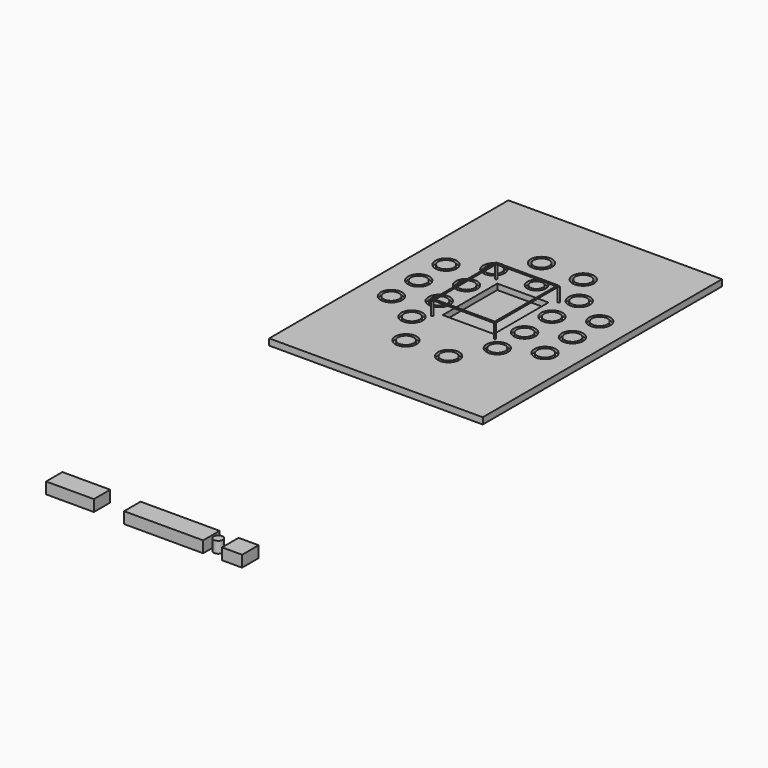
from build123d import *

# Parameters (mm, degrees)
F0_W      = 22860
F0_H      = 32004
F1_DEPTH  = 25.4
F2_W      = 5486.4
F2_H      = 7315.2
F3_DEPTH  = 76.2
F2_R      = 838.2
F4_DEPTH  = 685.8
F2_R_2    = 685.8
F2_R_3    = 844.55
F2_W_2    = 22872.7
F2_H_2    = 32016.7
F2_R_4    = 1143
F2_R_5    = 101.6
F2_R_6    = 1149.35
F2_R_7    = 990.6
F5_DEPTH  = 355.6
F6_DEPTH  = 2133.6
F8_W      = 6705.6
F8_H      = 8534.4
F8_W_2    = 6502.4
F8_H_2    = 8331.2
F9_DEPTH  = 101.6
F10_W     = 5118.2244420052
F10_H     = 2182.9090118408
F11_DEPTH = 1219.2
F10_W_2   = 8467.0696258545
F10_H_2   = 2208.8012695312
F10_W_3   = 2147.4456787109
F10_R     = 490.8447265625


# Not quite as in the source:
# - a feature names something its author has since deleted; it is built from what else it names


with BuildPart() as f1:
    # F0 (on Top) → F1 (new body)
    with BuildSketch(Plane.XY):
        with Locations((11430, 16002)):
            Rectangle(F0_W, F0_H)
    extrude(amount=F1_DEPTH)

    # F2 (on Top) → F6 (join)
    with BuildSketch(Plane.XY):
        with Locations((8077.2, 20269.2)):
            Circle(F2_R_5)
        with Locations((14782.8, 20269.2)):
            Circle(F2_R_5)
        with Locations((8077.2, 11734.8)):
            Circle(F2_R_5)
        with Locations((14782.8, 11734.8)):
            Circle(F2_R_5)
    extrude(amount=F6_DEPTH)

    # F8 (on offset) → F9 (join)
    with BuildSketch(Plane.XY.offset(2133.6)):
        with Locations((11430, 16002)):
            Rectangle(F8_W, F8_H)
        with Locations((11430, 16002)):
            Rectangle(F8_W_2, F8_H_2, mode=Mode.SUBTRACT)
    extrude(amount=F9_DEPTH)


with BuildPart() as f3:
    # F2 (on Top) → F3 (new body)
    with BuildSketch(Plane.XY):
        with Locations((11430, 16002)):
            Rectangle(F2_W, F2_H)
    extrude(amount=F3_DEPTH)


with BuildPart() as f4:
    # F2 (on Top) → F4 (new body)
    with BuildSketch(Plane.XY):
        with Locations((3200.4, 12344.4)):
            Circle(F2_R)
    extrude(amount=F4_DEPTH)


with BuildPart() as f4b:
    # F2 (on Top) → F4, piece 2 (new body)
    with BuildSketch(Plane.XY):
        with Locations((3200.4, 16002)):
            Circle(F2_R)
    extrude(amount=F4_DEPTH)


with BuildPart() as f4c:
    # F2 (on Top) → F4, piece 3 (new body)
    with BuildSketch(Plane.XY):
        with Locations((3200.4, 19659.6)):
            Circle(F2_R)
    extrude(amount=F4_DEPTH)


with BuildPart() as f4d:
    # F2 (on Top) → F4, piece 4 (new body)
    with BuildSketch(Plane.XY):
        with Locations((6858, 21488.4)):
            Circle(F2_R)
    extrude(amount=F4_DEPTH)


with BuildPart() as f4e:
    # F2 (on Top) → F4, piece 5 (new body)
    with BuildSketch(Plane.XY):
        with Locations((11430, 21488.4)):
            Circle(F2_R_2)
    extrude(amount=F4_DEPTH)


with BuildPart() as f4f:
    # F2 (on Top) → F4, piece 6 (new body)
    with BuildSketch(Plane.XY):
        with Locations((16002, 21488.4)):
            Circle(F2_R)
    extrude(amount=F4_DEPTH)


with BuildPart() as f4g:
    # F2 (on Top) → F4, piece 7 (new body)
    with BuildSketch(Plane.XY):
        with Locations((19659.6, 19659.6)):
            Circle(F2_R)
    extrude(amount=F4_DEPTH)


with BuildPart() as f4h:
    # F2 (on Top) → F4, piece 8 (new body)
    with BuildSketch(Plane.XY):
        with Locations((19659.6, 16002)):
            Circle(F2_R)
    extrude(amount=F4_DEPTH)


with BuildPart() as f4i:
    # F2 (on Top) → F4, piece 9 (new body)
    with BuildSketch(Plane.XY):
        with Locations((16002, 17830.8)):
            Circle(F2_R)
    extrude(amount=F4_DEPTH)


with BuildPart() as f4j:
    # F2 (on Top) → F4, piece 10 (new body)
    with BuildSketch(Plane.XY):
        with Locations((16002, 14173.2)):
            Circle(F2_R)
    extrude(amount=F4_DEPTH)


with BuildPart() as f4k:
    # F2 (on Top) → F4, piece 11 (new body)
    with BuildSketch(Plane.XY):
        with Locations((19659.6, 12344.4)):
            Circle(F2_R)
    extrude(amount=F4_DEPTH)


with BuildPart() as f4l:
    # F2 (on Top) → F4, piece 12 (new body)
    with BuildSketch(Plane.XY):
        with Locations((16002, 10515.6)):
            Circle(F2_R)
    extrude(amount=F4_DEPTH)


with BuildPart() as f4m:
    # F2 (on Top) → F4, piece 13 (new body)
    with BuildSketch(Plane.XY):
        with Locations((13716, 6858)):
            Circle(F2_R)
    extrude(amount=F4_DEPTH)


with BuildPart() as f4n:
    # F2 (on Top) → F4, piece 14 (new body)
    with BuildSketch(Plane.XY):
        with Locations((9144, 6858)):
            Circle(F2_R)
    extrude(amount=F4_DEPTH)


with BuildPart() as f4o:
    # F2 (on Top) → F4, piece 15 (new body)
    with BuildSketch(Plane.XY):
        with Locations((6858, 10515.6)):
            Circle(F2_R)
    extrude(amount=F4_DEPTH)


with BuildPart() as f4p:
    # F2 (on Top) → F4, piece 16 (new body)
    with BuildSketch(Plane.XY):
        with Locations((6858, 14173.2)):
            Circle(F2_R_3)
    extrude(amount=F4_DEPTH)


with BuildPart() as f4q:
    # F2 (on Top) → F4, piece 17 (new body)
    with BuildSketch(Plane.XY):
        with Locations((6858, 17830.8)):
            Circle(F2_R)
    extrude(amount=F4_DEPTH)


with BuildPart() as f4r:
    # F2 (on Top) → F4, piece 18 (new body)
    with BuildSketch(Plane.XY):
        with Locations((9253.4654006958, 24868.1221923828)):
            Circle(F2_R)
    extrude(amount=F4_DEPTH)


with BuildPart() as f4s:
    # F2 (on Top) → F4, piece 19 (new body)
    with BuildSketch(Plane.XY):
        with Locations((13846.1694717407, 24722.4292755127)):
            Circle(F2_R)
    extrude(amount=F4_DEPTH)


with BuildPart() as f4t:
    # F2 (on Top) → F4, piece 20 (new body)
    with BuildSketch(Plane.XY):
        with Locations((11430, 16002)):
            Rectangle(F2_W_2, F2_H_2)
        with Locations((9144, 6858)):
            Circle(F2_R_4, mode=Mode.SUBTRACT)
        with Locations((3200.4, 12344.4)):
            Circle(F2_R_4, mode=Mode.SUBTRACT)
        with Locations((6858, 10515.6)):
            Circle(F2_R_4, mode=Mode.SUBTRACT)
        with Locations((8077.2, 11734.8)):
            Circle(F2_R_5, mode=Mode.SUBTRACT)
        with Locations((6858, 14173.2)):
            Circle(F2_R_6, mode=Mode.SUBTRACT)
        with Locations((13716, 6858)):
            Circle(F2_R_4, mode=Mode.SUBTRACT)
        with Locations((14782.8, 11734.8)):
            Circle(F2_R_5, mode=Mode.SUBTRACT)
        with Locations((16002, 10515.6)):
            Circle(F2_R_4, mode=Mode.SUBTRACT)
        with Locations((16002, 14173.2)):
            Circle(F2_R_6, mode=Mode.SUBTRACT)
        with Locations((19659.6, 12344.4)):
            Circle(F2_R_4, mode=Mode.SUBTRACT)
        with Locations((3200.4, 16002)):
            Circle(F2_R_4, mode=Mode.SUBTRACT)
        with Locations((3200.4, 19659.6)):
            Circle(F2_R_4, mode=Mode.SUBTRACT)
        with Locations((6858, 17830.8)):
            Circle(F2_R_4, mode=Mode.SUBTRACT)
        with Locations((6858, 21488.4)):
            Circle(F2_R_4, mode=Mode.SUBTRACT)
        with Locations((8077.2, 20269.2)):
            Circle(F2_R_5, mode=Mode.SUBTRACT)
        with Locations((9253.4654006958, 24868.1221923828)):
            Circle(F2_R_4, mode=Mode.SUBTRACT)
        with Locations((11430, 16002)):
            Rectangle(F2_W, F2_H, mode=Mode.SUBTRACT)
        with Locations((16002, 17830.8)):
            Circle(F2_R_4, mode=Mode.SUBTRACT)
        with Locations((11430, 21488.4)):
            Circle(F2_R_7, mode=Mode.SUBTRACT)
        with Locations((14782.8, 20269.2)):
            Circle(F2_R_5, mode=Mode.SUBTRACT)
        with Locations((16002, 21488.4)):
            Circle(F2_R_4, mode=Mode.SUBTRACT)
        with Locations((19659.6, 16002)):
            Circle(F2_R_4, mode=Mode.SUBTRACT)
        with Locations((19659.6, 19659.6)):
            Circle(F2_R_4, mode=Mode.SUBTRACT)
        with Locations((13846.1694717407, 24722.4292755127)):
            Circle(F2_R_4, mode=Mode.SUBTRACT)
    extrude(amount=F4_DEPTH)


with BuildPart() as f5:
    # F2 (on Top) → F5 (new body)
    with BuildSketch(Plane.XY):
        with Locations((9144, 6858)):
            Circle(F2_R_4)
        with Locations((9144, 6858)):
            Circle(F2_R, mode=Mode.SUBTRACT)
    extrude(amount=F5_DEPTH)


with BuildPart() as f5b:
    # F2 (on Top) → F5, piece 2 (new body)
    with BuildSketch(Plane.XY):
        with Locations((6858, 10515.6)):
            Circle(F2_R_4)
        with Locations((6858, 10515.6)):
            Circle(F2_R, mode=Mode.SUBTRACT)
    extrude(amount=F5_DEPTH)


with BuildPart() as f5c:
    # F2 (on Top) → F5, piece 3 (new body)
    with BuildSketch(Plane.XY):
        with Locations((3200.4, 12344.4)):
            Circle(F2_R_4)
        with Locations((3200.4, 12344.4)):
            Circle(F2_R, mode=Mode.SUBTRACT)
    extrude(amount=F5_DEPTH)


with BuildPart() as f5d:
    # F2 (on Top) → F5, piece 4 (new body)
    with BuildSketch(Plane.XY):
        with Locations((3200.4, 16002)):
            Circle(F2_R_4)
        with Locations((3200.4, 16002)):
            Circle(F2_R, mode=Mode.SUBTRACT)
    extrude(amount=F5_DEPTH)


with BuildPart() as f5e:
    # F2 (on Top) → F5, piece 5 (new body)
    with BuildSketch(Plane.XY):
        with Locations((3200.4, 19659.6)):
            Circle(F2_R_4)
        with Locations((3200.4, 19659.6)):
            Circle(F2_R, mode=Mode.SUBTRACT)
    extrude(amount=F5_DEPTH)


with BuildPart() as f5f:
    # F2 (on Top) → F5, piece 6 (new body)
    with BuildSketch(Plane.XY):
        with Locations((6858, 21488.4)):
            Circle(F2_R_4)
        with Locations((6858, 21488.4)):
            Circle(F2_R, mode=Mode.SUBTRACT)
    extrude(amount=F5_DEPTH)


with BuildPart() as f5g:
    # F2 (on Top) → F5, piece 7 (new body)
    with BuildSketch(Plane.XY):
        with Locations((11430, 21488.4)):
            Circle(F2_R_7)
        with Locations((11430, 21488.4)):
            Circle(F2_R_2, mode=Mode.SUBTRACT)
    extrude(amount=F5_DEPTH)


with BuildPart() as f5h:
    # F2 (on Top) → F5, piece 8 (new body)
    with BuildSketch(Plane.XY):
        with Locations((16002, 21488.4)):
            Circle(F2_R_4)
        with Locations((16002, 21488.4)):
            Circle(F2_R, mode=Mode.SUBTRACT)
    extrude(amount=F5_DEPTH)


with BuildPart() as f5i:
    # F2 (on Top) → F5, piece 9 (new body)
    with BuildSketch(Plane.XY):
        with Locations((16002, 17830.8)):
            Circle(F2_R_4)
        with Locations((16002, 17830.8)):
            Circle(F2_R, mode=Mode.SUBTRACT)
    extrude(amount=F5_DEPTH)


with BuildPart() as f5j:
    # F2 (on Top) → F5, piece 10 (new body)
    with BuildSketch(Plane.XY):
        with Locations((19659.6, 19659.6)):
            Circle(F2_R_4)
        with Locations((19659.6, 19659.6)):
            Circle(F2_R, mode=Mode.SUBTRACT)
    extrude(amount=F5_DEPTH)


with BuildPart() as f5k:
    # F2 (on Top) → F5, piece 11 (new body)
    with BuildSketch(Plane.XY):
        with Locations((16002, 14173.2)):
            Circle(F2_R_6)
        with Locations((16002, 14173.2)):
            Circle(F2_R_3, mode=Mode.SUBTRACT)
    extrude(amount=F5_DEPTH)


with BuildPart() as f5l:
    # F2 (on Top) → F5, piece 12 (new body)
    with BuildSketch(Plane.XY):
        with Locations((19659.6, 16002)):
            Circle(F2_R_4)
        with Locations((19659.6, 16002)):
            Circle(F2_R, mode=Mode.SUBTRACT)
    extrude(amount=F5_DEPTH)


with BuildPart() as f5m:
    # F2 (on Top) → F5, piece 13 (new body)
    with BuildSketch(Plane.XY):
        with Locations((19659.6, 12344.4)):
            Circle(F2_R_4)
        with Locations((19659.6, 12344.4)):
            Circle(F2_R, mode=Mode.SUBTRACT)
    extrude(amount=F5_DEPTH)


with BuildPart() as f5n:
    # F2 (on Top) → F5, piece 14 (new body)
    with BuildSketch(Plane.XY):
        with Locations((16002, 10515.6)):
            Circle(F2_R_4)
        with Locations((16002, 10515.6)):
            Circle(F2_R, mode=Mode.SUBTRACT)
    extrude(amount=F5_DEPTH)


with BuildPart() as f5o:
    # F2 (on Top) → F5, piece 15 (new body)
    with BuildSketch(Plane.XY):
        with Locations((13716, 6858)):
            Circle(F2_R_4)
        with Locations((13716, 6858)):
            Circle(F2_R_3, mode=Mode.SUBTRACT)
    extrude(amount=F5_DEPTH)


with BuildPart() as f5p:
    # F2 (on Top) → F5, piece 16 (new body)
    with BuildSketch(Plane.XY):
        with Locations((6858, 14173.2)):
            Circle(F2_R_6)
        with Locations((6858, 14173.2)):
            Circle(F2_R_3, mode=Mode.SUBTRACT)
    extrude(amount=F5_DEPTH)


with BuildPart() as f5q:
    # F2 (on Top) → F5, piece 17 (new body)
    with BuildSketch(Plane.XY):
        with Locations((6858, 17830.8)):
            Circle(F2_R_4)
        with Locations((6858, 17830.8)):
            Circle(F2_R, mode=Mode.SUBTRACT)
    extrude(amount=F5_DEPTH)


with BuildPart() as f11:
    # F10 (on face) → F11 (new body)
    with BuildSketch(Plane(origin=(0, 0, 0), x_dir=(1, 0, 0), z_dir=(0, 0, -1))):
        with Locations((3349.4084775448, 29780.2495956421)):
            Rectangle(F10_W, F10_H)
    extrude(amount=F11_DEPTH)


with BuildPart() as f11b:
    # F10 (on face) → F11, piece 2 (new body)
    with BuildSketch(Plane(origin=(0, 0, 0), x_dir=(1, 0, 0), z_dir=(0, 0, -1))):
        with Locations((13477.9901504517, 29891.6168212891)):
            Rectangle(F10_W_2, F10_H_2)
    extrude(amount=F11_DEPTH)


with BuildPart() as f11c:
    # F10 (on face) → F11, piece 3 (new body)
    with BuildSketch(Plane(origin=(0, 0, 0), x_dir=(1, 0, 0), z_dir=(0, 0, -1))):
        with Locations((20809.9822998047, 29891.6168212891)):
            Rectangle(F10_W_3, F10_H_2)
    extrude(amount=F11_DEPTH)


with BuildPart() as f11d:
    # F10 (on face) → F11, piece 4 (new body)
    with BuildSketch(Plane(origin=(0, 0, 0), x_dir=(1, 0, 0), z_dir=(0, 0, -1))):
        with Locations((18447.7920532227, 29891.6168212891)):
            Circle(F10_R)
    extrude(amount=F11_DEPTH)


solid = Compound([f1.part, f3.part, f4.part, f4b.part, f4c.part, f4d.part, f4e.part, f4f.part, f4g.part, f4h.part, f4i.part, f4j.part, f4k.part, f4l.part, f4m.part, f4n.part, f4o.part, f4p.part, f4q.part, f4r.part, f4s.part, f4t.part, f5.part, f5b.part, f5c.part, f5d.part, f5e.part, f5f.part, f5g.part, f5h.part, f5i.part, f5j.part, f5k.part, f5l.part, f5m.part, f5n.part, f5o.part, f5p.part, f5q.part, f11.part, f11b.part, f11c.part, f11d.part])
